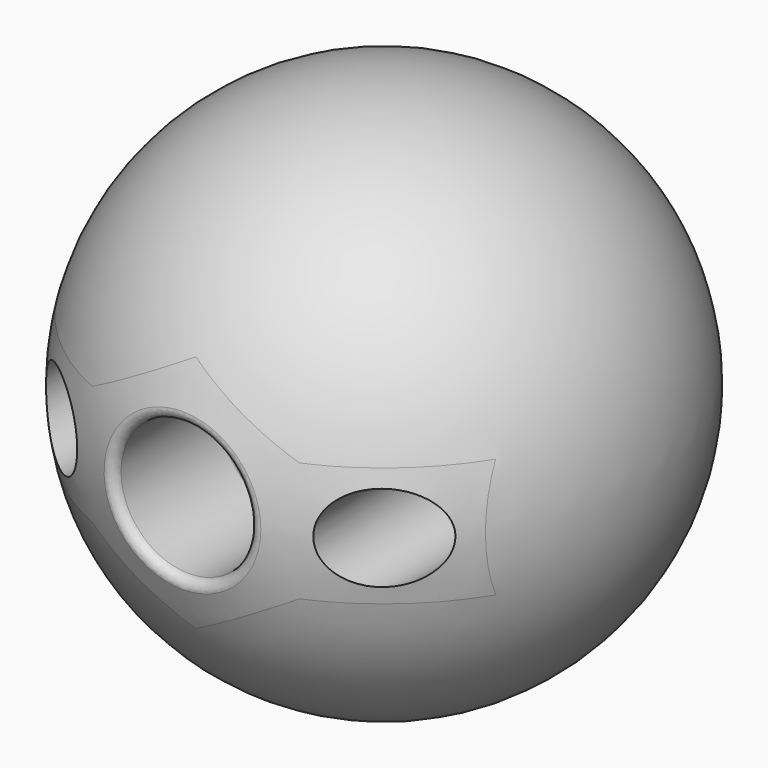
from build123d import *

# Parameters (mm, degrees)
F2_DEPTH  = 20.5
F3_W      = 7
F3_H      = 7.25
F3_R      = 1.5
F4_DEPTH  = 25
F5_R      = 1.5
F6_DEPTH  = 25
F3_R_2    = 4.1
F7_DEPTH  = 5
F9_DEPTH  = 25
F11_R     = 2.625
F11_R_2   = 1.5
F12_DEPTH = 25
F13_DEPTH = 5.5
F14_R     = 0.5
F11_R_3   = 4.1
F15_DEPTH = 6.8
F16_R     = 1
F17_R     = 0.5


with BuildPart() as f1:
    # F0 (on Top) → F1 (revolve)
    with BuildSketch(Plane.XY):
        with BuildLine():
            Line((0, -15.4657686521), (4.1, -15.4657686521))
            ThreePointArc((4.1, -15.4657686521), (15.8658800328, 2.0673293843), (0, 16))
            Line((0, 16), (0, -15.4657686521))
        make_face()
    revolve(axis=Axis((0, 0.267115674, 0), (0, 1, 0)))

    # F2 (cut): a face of the model
    f2_faces = [f1.faces().sort_by_distance(p)[0] for p in [
        (0, -15.4657686521, 0),
    ]]
    extrude(f2_faces, amount=-F2_DEPTH, mode=Mode.SUBTRACT)

    # F3 (on face) → F4 (join)
    with BuildSketch(Plane.XZ.offset(-5.0342313479)):
        Polygon((6.2786841774, 3.625), (0, 7.25), (-6.2786841774, 3.625), (-6.2786841774, -3.625), (0, -7.25), (6.2786841774, -3.625), align=None)
        with Locations((-9.7786841774, 0)):
            Rectangle(F3_W, F3_H)
        with Locations((-9.7786841774, 0)):
            Circle(F3_R, mode=Mode.SUBTRACT)
        with Locations((9.7786841774, 0)):
            Rectangle(F3_W, F3_H)
        with Locations((9.7786841774, 0)):
            Circle(F3_R, mode=Mode.SUBTRACT)
    extrude(amount=F4_DEPTH)

    # F5 (on face) → F6 (cut)
    with BuildSketch(Plane.XZ.offset(19.9657686521)):
        Polygon((13.2786841774, 3.625), (6.2786841774, 3.625), (0, 7.25), (-6.2786841774, 3.625), (-13.2786841774, 3.625), (-13.2786841774, -3.625), (-6.2786841774, -3.625), (0, -7.25), (6.2786841774, -3.625), (13.2786841774, -3.625), align=None)
        with Locations((-9.7786841774, 0)):
            Circle(F5_R, mode=Mode.SUBTRACT)
        with Locations((9.7786841774, 0)):
            Circle(F5_R, mode=Mode.SUBTRACT)
        with Locations((-9.7786841774, 0)):
            Circle(F5_R)
        with Locations((9.7786841774, 0)):
            Circle(F5_R)
    extrude(amount=-F6_DEPTH, mode=Mode.SUBTRACT)

    # F3 (on face) → F7 (join)
    with BuildSketch(Plane.XZ.offset(-5.0342313479)):
        Polygon((6.2786841774, 3.625), (0, 7.25), (-6.2786841774, 3.625), (-6.2786841774, -3.625), (0, -7.25), (6.2786841774, -3.625), align=None)
        Circle(F3_R_2, mode=Mode.SUBTRACT)
        with Locations((-9.7786841774, 0)):
            Rectangle(F3_W, F3_H)
        with Locations((-9.7786841774, 0)):
            Circle(F3_R, mode=Mode.SUBTRACT)
        with Locations((9.7786841774, 0)):
            Rectangle(F3_W, F3_H)
        with Locations((9.7786841774, 0)):
            Circle(F3_R, mode=Mode.SUBTRACT)
    extrude(amount=F7_DEPTH)


with BuildPart() as f9:
    # F9 (new): a face of the model
    f9_faces = [f1.part.faces().sort_by_distance(p)[0] for p in [
        (2.9880523159, 0.0342313479, 5.1754584269),
    ]]
    extrude(f9_faces, amount=F9_DEPTH)

    # F8 (on Top) → F10 (revolve, cut)
    with BuildSketch(Plane.XY):
        with BuildLine():
            ThreePointArc((0, 16), (11.313708499, 11.313708499), (16, 0))
            ThreePointArc((16, 0), (11.313708499, -11.313708499), (0, -16))
            Line((0, -16), (0, -32.4343107641))
            Line((0, -32.4343107641), (22.5159879774, -32.4343107641))
            Line((22.5159879774, -32.4343107641), (22.5159879774, 32.4343107641))
            Line((22.5159879774, 32.4343107641), (0, 32.4343107641))
            Line((0, 32.4343107641), (0, 16))
        make_face()
    revolve(axis=Axis((0, 0, 0), (0, 1, 0)), mode=Mode.SUBTRACT)

    # F11 (on face) → F12 (cut)
    with BuildSketch(Plane(origin=(0, 0.0342313479, 0), x_dir=(-1, 0, 0), z_dir=(0, 1, 0))):
        with Locations((-9.7786841774, 0)):
            Circle(F11_R)
        with Locations((-9.7786841774, 0)):
            Circle(F11_R_2, mode=Mode.SUBTRACT)
        with Locations((9.7786841774, 0)):
            Circle(F11_R)
        with Locations((9.7786841774, 0)):
            Circle(F11_R_2, mode=Mode.SUBTRACT)
    extrude(amount=-F12_DEPTH, mode=Mode.SUBTRACT)

    # F11 (on face) → F13 (join)
    with BuildSketch(Plane(origin=(0, 0.0342313479, 0), x_dir=(-1, 0, 0), z_dir=(0, 1, 0))):
        with Locations((-9.7786841774, 0)):
            Circle(F11_R)
        with Locations((-9.7786841774, 0)):
            Circle(F11_R_2, mode=Mode.SUBTRACT)
        with Locations((9.7786841774, 0)):
            Circle(F11_R)
        with Locations((9.7786841774, 0)):
            Circle(F11_R_2, mode=Mode.SUBTRACT)
    extrude(amount=-F13_DEPTH)

    # F14
    f14_edges = [f9.edges().sort_by_distance(p)[0] for p in [
        (-4.1, -15.465769, 0),
    ]]
    fillet(f14_edges, radius=F14_R)

    # F11 (on face) → F15 (cut)
    with BuildSketch(Plane(origin=(0, 0.0342313479, 0), x_dir=(-1, 0, 0), z_dir=(0, 1, 0))):
        Polygon((-6.2786841774, 3.625), (-6.2786841774, -3.625), (0, -7.25), (6.2786841774, -3.625), (6.2786841774, 3.625), (0, 7.25), align=None)
        Circle(F11_R_3, mode=Mode.SUBTRACT)
    extrude(amount=-F15_DEPTH, mode=Mode.SUBTRACT)

    # F16
    f16_edges = [f9.edges().sort_by_distance(p)[0] for p in [
        (13.278684, 0.034231, 0),
        (9.778684, 0.034231, -3.625),
        (6.278684, 0.034231, 0),
        (9.778684, 0.034231, 3.625),
        (-6.278684, 0.034231, 0),
        (-9.778684, 0.034231, 3.625),
        (-13.278684, 0.034231, 0),
        (-9.778684, 0.034231, -3.625),
        (-3.139342, -6.765769, 5.4375),
        (3.139342, -6.765769, -5.4375),
        (-3.139342, -6.765769, -5.4375),
        (3.139342, -6.765769, 5.4375),
    ]]
    fillet(f16_edges, radius=F16_R)

    # F17
    f17_edges = [f9.edges().sort_by_distance(p)[0] for p in [
        (-4.1, -6.765769, 0),
    ]]
    fillet(f17_edges, radius=F17_R)


solid = Compound([f1.part, f9.part])
